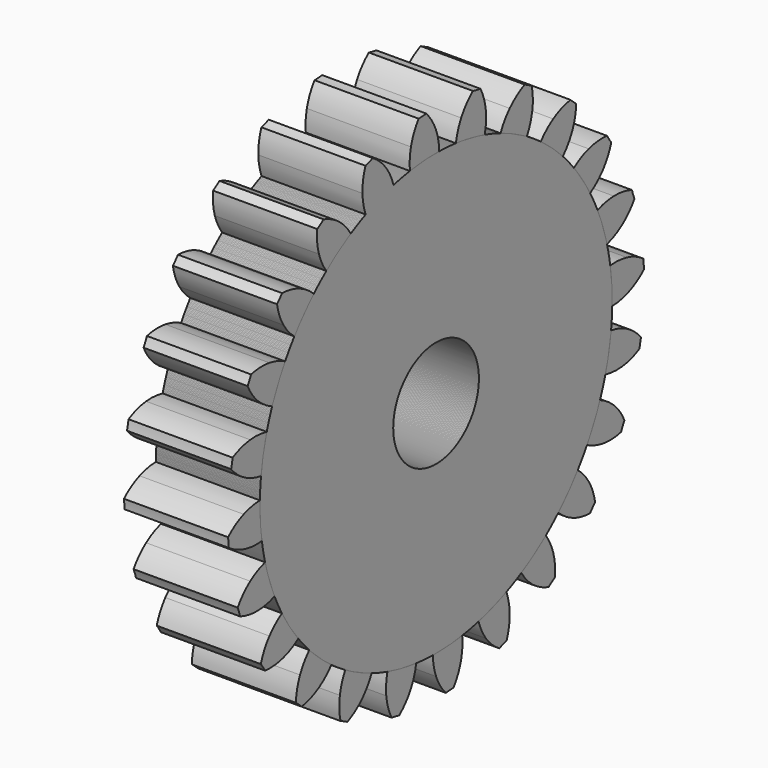
from build123d import *

# Parameters (mm, degrees)
F0_R     = 13.081
F1_DEPTH = 25.4
F2_COUNT = 24
F2_ANGLE = 345


with BuildPart() as f1:
    # F0 (on Right) → F1 (new body)
    with BuildSketch(Plane.YZ):
        with BuildLine():
            ThreePointArc((53.721, 0), (38.329016413, 37.6408334368), (0.9731977694, 53.7121841587))
            ThreePointArc((0.9731977694, 53.7121841587), (-3.5135215054, 53.6059792153), (-7.9757188017, 53.1256411782))
            ThreePointArc((-7.9757188017, 53.1256411782), (-35.0534039093, -40.7087793402), (53.721, 0))
        make_face()
        Circle(F0_R, mode=Mode.SUBTRACT)
        with BuildLine():
            ThreePointArc((-7.6584938023, 58.1720357962), (-3.8374632044, 58.5483744621), (0, 58.674))
            ThreePointArc((0, 58.674), (-1.2621662791, 61.1979128197), (-2.9892332778, 63.4296025875))
            ThreePointArc((-2.9892332778, 63.4296025875), (-4.1501638482, 63.3192643466), (-5.315564527, 63.2771267818))
            ThreePointArc((-5.315564527, 63.2771267818), (-6.7365622606, 60.8391019503), (-7.6584938023, 58.1720357962))
        make_face()
        with BuildLine():
            ThreePointArc((0.9731977694, 53.7121841587), (0.7012174063, 56.235186803), (0, 58.674))
            ThreePointArc((0, 58.674), (-3.8374632044, 58.5483744621), (-7.6584938023, 58.1720357962))
            ThreePointArc((-7.6584938023, 58.1720357962), (-8.0353831964, 55.6625597463), (-7.9757188017, 53.1256411782))
            ThreePointArc((-7.9757188017, 53.1256411782), (-3.5135215054, 53.6059792153), (0.9731977694, 53.7121841587))
        make_face()
    extrude(amount=F1_DEPTH)


with BuildPart() as f2_1:
    # F2: instance of F1
    add(f1.part.rotate(Axis((0, 0, 0), (-1, 0, 0)), 1 * F2_ANGLE / (F2_COUNT - 1)))


with BuildPart() as f2_2:
    # F2: instance of F1
    add(f1.part.rotate(Axis((0, 0, 0), (-1, 0, 0)), 2 * F2_ANGLE / (F2_COUNT - 1)))


with BuildPart() as f2_3:
    # F2: instance of F1
    add(f1.part.rotate(Axis((0, 0, 0), (-1, 0, 0)), 3 * F2_ANGLE / (F2_COUNT - 1)))


with BuildPart() as f2_4:
    # F2: instance of F1
    add(f1.part.rotate(Axis((0, 0, 0), (-1, 0, 0)), 4 * F2_ANGLE / (F2_COUNT - 1)))


with BuildPart() as f2_5:
    # F2: instance of F1
    add(f1.part.rotate(Axis((0, 0, 0), (-1, 0, 0)), 5 * F2_ANGLE / (F2_COUNT - 1)))


with BuildPart() as f2_6:
    # F2: instance of F1
    add(f1.part.rotate(Axis((0, 0, 0), (-1, 0, 0)), 6 * F2_ANGLE / (F2_COUNT - 1)))


with BuildPart() as f2_7:
    # F2: instance of F1
    add(f1.part.rotate(Axis((0, 0, 0), (-1, 0, 0)), 7 * F2_ANGLE / (F2_COUNT - 1)))


with BuildPart() as f2_8:
    # F2: instance of F1
    add(f1.part.rotate(Axis((0, 0, 0), (-1, 0, 0)), 8 * F2_ANGLE / (F2_COUNT - 1)))


with BuildPart() as f2_9:
    # F2: instance of F1
    add(f1.part.rotate(Axis((0, 0, 0), (-1, 0, 0)), 9 * F2_ANGLE / (F2_COUNT - 1)))


with BuildPart() as f2_10:
    # F2: instance of F1
    add(f1.part.rotate(Axis((0, 0, 0), (-1, 0, 0)), 10 * F2_ANGLE / (F2_COUNT - 1)))


with BuildPart() as f2_11:
    # F2: instance of F1
    add(f1.part.rotate(Axis((0, 0, 0), (-1, 0, 0)), 11 * F2_ANGLE / (F2_COUNT - 1)))


with BuildPart() as f2_12:
    # F2: instance of F1
    add(f1.part.rotate(Axis((0, 0, 0), (-1, 0, 0)), 12 * F2_ANGLE / (F2_COUNT - 1)))


with BuildPart() as f2_13:
    # F2: instance of F1
    add(f1.part.rotate(Axis((0, 0, 0), (-1, 0, 0)), 13 * F2_ANGLE / (F2_COUNT - 1)))


with BuildPart() as f2_14:
    # F2: instance of F1
    add(f1.part.rotate(Axis((0, 0, 0), (-1, 0, 0)), 14 * F2_ANGLE / (F2_COUNT - 1)))


with BuildPart() as f2_15:
    # F2: instance of F1
    add(f1.part.rotate(Axis((0, 0, 0), (-1, 0, 0)), 15 * F2_ANGLE / (F2_COUNT - 1)))


with BuildPart() as f2_16:
    # F2: instance of F1
    add(f1.part.rotate(Axis((0, 0, 0), (-1, 0, 0)), 16 * F2_ANGLE / (F2_COUNT - 1)))


with BuildPart() as f2_17:
    # F2: instance of F1
    add(f1.part.rotate(Axis((0, 0, 0), (-1, 0, 0)), 17 * F2_ANGLE / (F2_COUNT - 1)))


with BuildPart() as f2_18:
    # F2: instance of F1
    add(f1.part.rotate(Axis((0, 0, 0), (-1, 0, 0)), 18 * F2_ANGLE / (F2_COUNT - 1)))


with BuildPart() as f2_19:
    # F2: instance of F1
    add(f1.part.rotate(Axis((0, 0, 0), (-1, 0, 0)), 19 * F2_ANGLE / (F2_COUNT - 1)))


with BuildPart() as f2_20:
    # F2: instance of F1
    add(f1.part.rotate(Axis((0, 0, 0), (-1, 0, 0)), 20 * F2_ANGLE / (F2_COUNT - 1)))


with BuildPart() as f2_21:
    # F2: instance of F1
    add(f1.part.rotate(Axis((0, 0, 0), (-1, 0, 0)), 21 * F2_ANGLE / (F2_COUNT - 1)))


with BuildPart() as f2_22:
    # F2: instance of F1
    add(f1.part.rotate(Axis((0, 0, 0), (-1, 0, 0)), 22 * F2_ANGLE / (F2_COUNT - 1)))


with BuildPart() as f2_23:
    # F2: instance of F1
    add(f1.part.rotate(Axis((0, 0, 0), (-1, 0, 0)), 23 * F2_ANGLE / (F2_COUNT - 1)))


solid = Compound([f1.part, f2_1.part, f2_2.part, f2_3.part, f2_4.part, f2_5.part, f2_6.part, f2_7.part, f2_8.part, f2_9.part, f2_10.part, f2_11.part, f2_12.part, f2_13.part, f2_14.part, f2_15.part, f2_16.part, f2_17.part, f2_18.part, f2_19.part, f2_20.part, f2_21.part, f2_22.part, f2_23.part])
